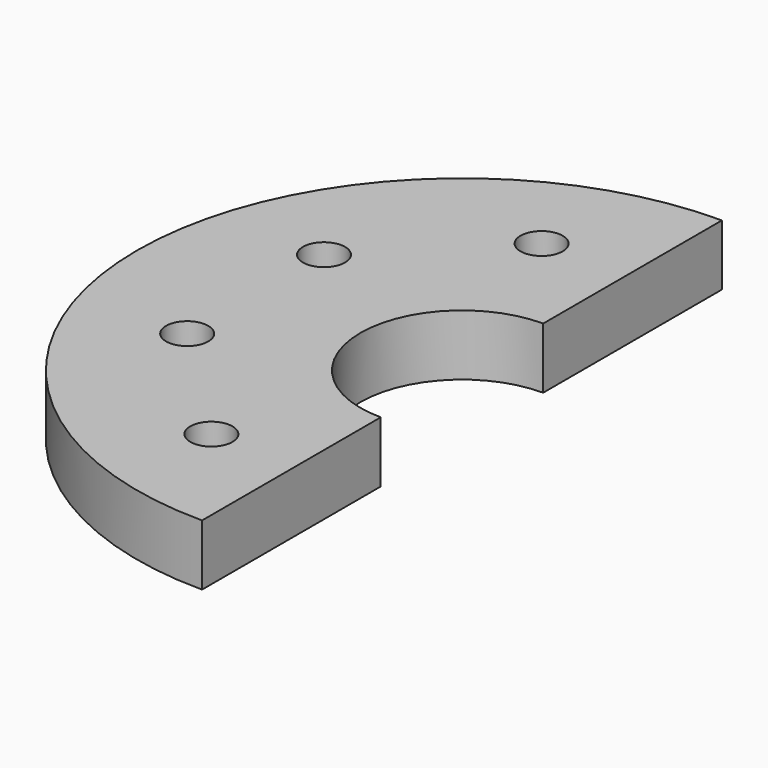
from build123d import *

# Parameters (mm, degrees)
F0_R     = 50.8
F1_DEPTH = 9.525
F2_R     = 15.875
F3_DEPTH = 9.526
F5_D     = 6.6
F6_R     = 3.3
F7_DEPTH = 9.526


with BuildPart() as f1:
    # F0 (on Top) → F1 (new body)
    with BuildSketch(Plane.XY):
        Circle(F0_R)
    extrude(amount=F1_DEPTH)

    # F2 (on face) → F3 (cut, through all)
    with BuildSketch(Plane.XY.offset(9.525)):
        Circle(F2_R)
    extrude(amount=-F3_DEPTH, mode=Mode.SUBTRACT)

    # F5 (through all)
    with Locations(Plane.XY.offset(9.525)):
        with Locations((-13.3652133, 32.2664949823), (-32.2664903636, 13.3652244507), (-32.2664949823, -13.3652133), (-13.3652244507, -32.2664903636), (13.3652133, -32.2664949823), (32.2664903636, -13.3652244507), (32.2664949823, 13.3652133), (13.3652244507, 32.2664903636)):
            Hole(F5_D / 2)

    # F6 (on face) → F7 (cut, through all)
    with BuildSketch(Plane.XY.offset(9.525)):
        with BuildLine():
            Line((92.0014753938, 88.4870588779), (0, 88.4870588779))
            Line((0, 88.4870588779), (0, 50.8))
            ThreePointArc((0, 50.8), (35.9210244843, 35.9210244843), (50.8, 0))
            ThreePointArc((50.8, 0), (35.9210244843, -35.9210244843), (0, -50.8))
            Line((0, -50.8), (0, -93.3939293027))
            Line((0, -93.3939293027), (92.0014753938, -93.3939293027))
            Line((92.0014753938, -93.3939293027), (92.0014753938, 88.4870588779))
        make_face()
        with BuildLine():
            ThreePointArc((50.8, 0), (35.9210244843, 35.9210244843), (0, 50.8))
            Line((0, 50.8), (0, 15.875))
            ThreePointArc((0, 15.875), (11.2253201513, 11.2253201513), (15.875, 0))
            ThreePointArc((15.875, 0), (11.2253201513, -11.2253201513), (0, -15.875))
            Line((0, -15.875), (0, -50.8))
            ThreePointArc((0, -50.8), (35.9210244843, -35.9210244843), (50.8, 0))
        make_face()
        with Locations((13.3652133, -32.2664949823)):
            Circle(F6_R, mode=Mode.SUBTRACT)
        with Locations((32.2664903636, -13.3652244507)):
            Circle(F6_R, mode=Mode.SUBTRACT)
        with Locations((13.3652244507, 32.2664903636)):
            Circle(F6_R, mode=Mode.SUBTRACT)
        with Locations((32.2664949823, 13.3652133)):
            Circle(F6_R, mode=Mode.SUBTRACT)
    extrude(amount=-F7_DEPTH, mode=Mode.SUBTRACT)


solid = f1.part
